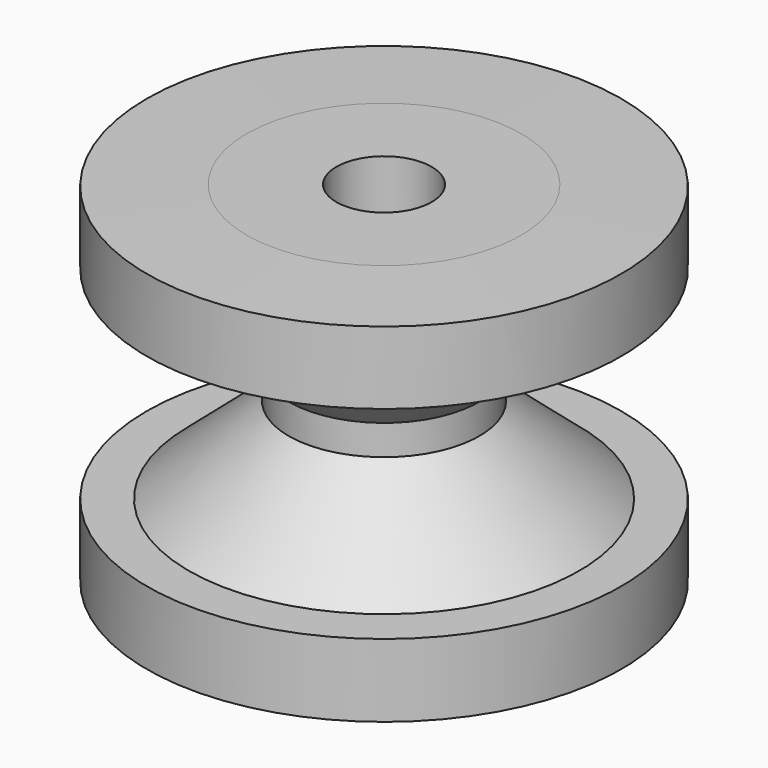
from build123d import *

# Parameters (mm, degrees)
F0_W        = 36.0753956601
F0_H        = 18.8608030145
F0_W_2      = 12.1251638026
F0_H_2      = 51.4777676715
F0_H_3      = 18.561429314
F2_C1_SIZE2 = 21.9075
F2_C1_SIZE  = 25.4
F2_C2_SIZE2 = 25.4
F2_C2_SIZE  = 21.9075
F4_SIZE2    = 25.4
F4_SIZE     = 0.41275


# Not quite as in the source:
# - a feature of the source that left no trace in its solid (it failed there, or was rolled back) is left out


with BuildPart() as f1:
    # F0 (on Front) → F1 (revolve)
    with BuildSketch(Plane.XZ):
        with Locations((-42.2873021699, 79.4695984927)):
            Rectangle(F0_W, F0_H)
        with Locations((-18.1870224386, 79.4695984927)):
            Rectangle(F0_W_2, F0_H)
        with Locations((-18.1870224386, 44.3003131497)):
            Rectangle(F0_W_2, F0_H_2)
        with Locations((-18.1870224386, 9.280714657)):
            Rectangle(F0_W_2, F0_H_3)
        with Locations((-42.2873021699, 9.280714657)):
            Rectangle(F0_W, F0_H_3)
    revolve(axis=Axis((0, 0, 53.2892593555), (0, 0, 1)))

    # F2: chamfer of 21.9075 x 25.4 on 2 edges, made by hand

    # F2_c1
    f2_c1_edges = [f1.edges().sort_by_distance(p)[0] for p in [
        (24.2496043399, 0, 70.0391969855),
    ]]
    f2_c1_side = f1.faces().sort_by_distance((24.6877543399, 0, 70.0391969855))[0]
    chamfer(f2_c1_edges, length=F2_C1_SIZE, length2=F2_C1_SIZE2, reference=f2_c1_side)

    # F2_c2
    f2_c2_edges = [f1.edges().sort_by_distance(p)[0] for p in [
        (24.2496043399, 0, 18.561429314),
    ]]
    f2_c2_side = f1.faces().sort_by_distance((24.2496043399, 0, 18.999579314))[0]
    chamfer(f2_c2_edges, length=F2_C2_SIZE, length2=F2_C2_SIZE2, reference=f2_c2_side)

    # F4
    f4_edges = [f1.edges().sort_by_distance(p)[0] for p in [
        (60.325, 0, 88.9),
    ]]
    chamfer(f4_edges, length=F4_SIZE, length2=F4_SIZE2)


solid = f1.part
